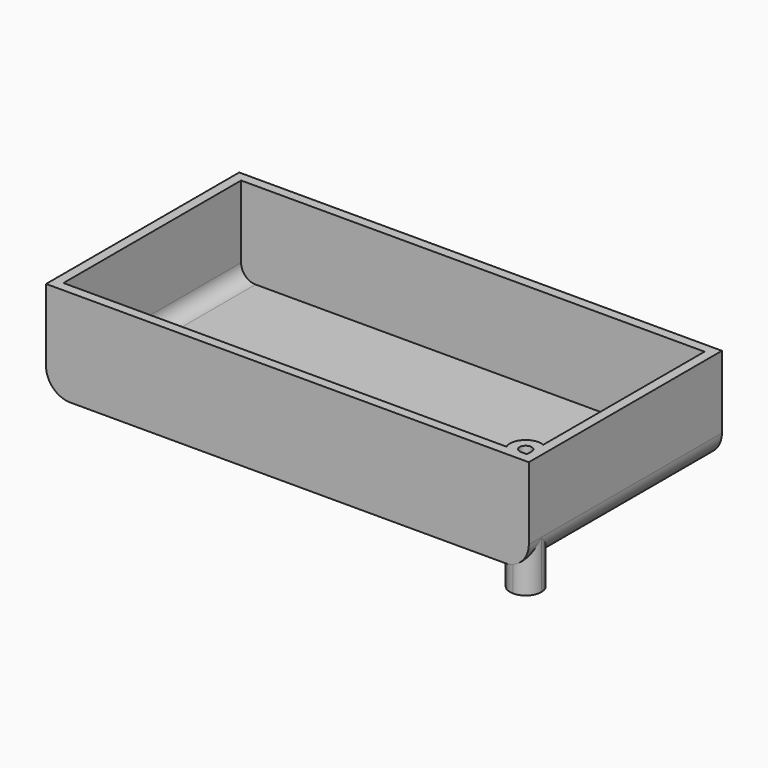
from build123d import *

# Parameters (mm, degrees)
F1_DEPTH = 25
F2_T     = -2
F4_DEPTH = 25


with BuildPart() as f1:
    # F0 (on Front) → F1 (new body, symmetric)
    with BuildSketch(Plane.XZ):
        with BuildLine():
            Line((50, 10), (-50, 10))
            Line((-50, 10), (-50, -5))
            ThreePointArc((-50, -5), (-48.5355339059, -8.5355339059), (-45, -10))
            Line((-45, -10), (45, -10))
            ThreePointArc((45, -10), (48.5355339059, -8.5355339059), (50, -5))
            Line((50, -5), (50, 10))
        make_face()
    extrude(amount=F1_DEPTH, both=True)

    # F2
    f2_openings = [f1.faces().sort_by_distance(p)[0] for p in [
        (0, 0, 10),
    ]]
    offset(amount=F2_T, openings=f2_openings)

    # F3 (on face) → F4 (join)
    with BuildSketch(Plane.XY.offset(10)):
        with BuildLine():
            Line((48, -18.7663880923), (48, -21.7598285526))
            Line((48, -21.7598285526), (48, -23))
            Line((48, -23), (46.7598285526, -23))
            Line((46.7598285526, -23), (43.7663880923, -23))
            ThreePointArc((43.7663880923, -23), (44.9597809557, -24.4539962641), (46.7598286169, -25))
            ThreePointArc((46.7598286169, -25), (49.050975778, -24.0509757325), (50, -21.7598285526))
            ThreePointArc((50, -21.7598285526), (49.4539962462, -19.959780929), (48, -18.7663880923))
        make_face()
        with BuildLine():
            ThreePointArc((46.7598285526, -23), (45.8828949123, -20.8828949123), (48, -21.7598285526))
            Line((48, -21.7598285526), (48, -18.7663880923))
            ThreePointArc((48, -18.7663880923), (44.4686813499, -19.4686813499), (43.7663880923, -23))
            Line((43.7663880923, -23), (46.7598285526, -23))
        make_face()
    extrude(amount=-F4_DEPTH)


solid = f1.part
